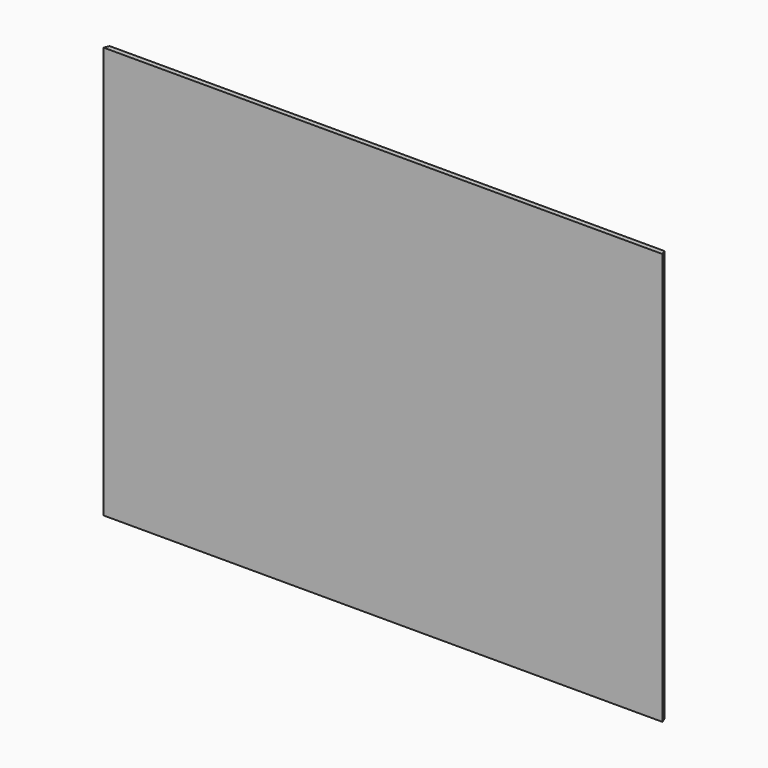
from build123d import *

# Parameters (mm, degrees)
F0_W       = 1429.9238244843
F0_H       = 1054.1
F1_DEPTH   = 12.7
F2_SIZE2   = 5.260502
F2_SIZE    = 12.69999
F2_2_SIZE2 = 5.260502
F2_2_SIZE  = 12.69999


# Not quite as in the source:
# - a fillet or chamfer is up to 0.001 mm smaller than in the source, because OpenCascade refuses the exact size


with BuildPart() as f1:
    # F0 (on Front) → F1 (new body)
    with BuildSketch(Plane.XZ):
        with Locations((714.9619122421, 527.05)):
            Rectangle(F0_W, F0_H)
    extrude(amount=-F1_DEPTH)

    # F2 (size 12.7 and 5.2605122421 in the source; OpenCascade refuses exactly that, so slightly less here)
    f2_edges = [f1.edges().sort_by_distance(p)[0] for p in [
        (1429.923824, 12.7, 527.05),
    ]]
    f2_side = f1.faces().sort_by_distance((1429.923824, 6.35, 527.05))[0]
    chamfer(f2_edges, length=F2_SIZE, length2=F2_SIZE2, reference=f2_side)

    # F2#2 (size 12.7 and 5.2605122421 in the source; OpenCascade refuses exactly that, so slightly less here)
    f2_2_edges = [f1.edges().sort_by_distance(p)[0] for p in [
        (0, 12.7, 527.05),
    ]]
    f2_2_side = f1.faces().sort_by_distance((0, 6.35, 527.05))[0]
    chamfer(f2_2_edges, length=F2_2_SIZE, length2=F2_2_SIZE2, reference=f2_2_side)


solid = f1.part
